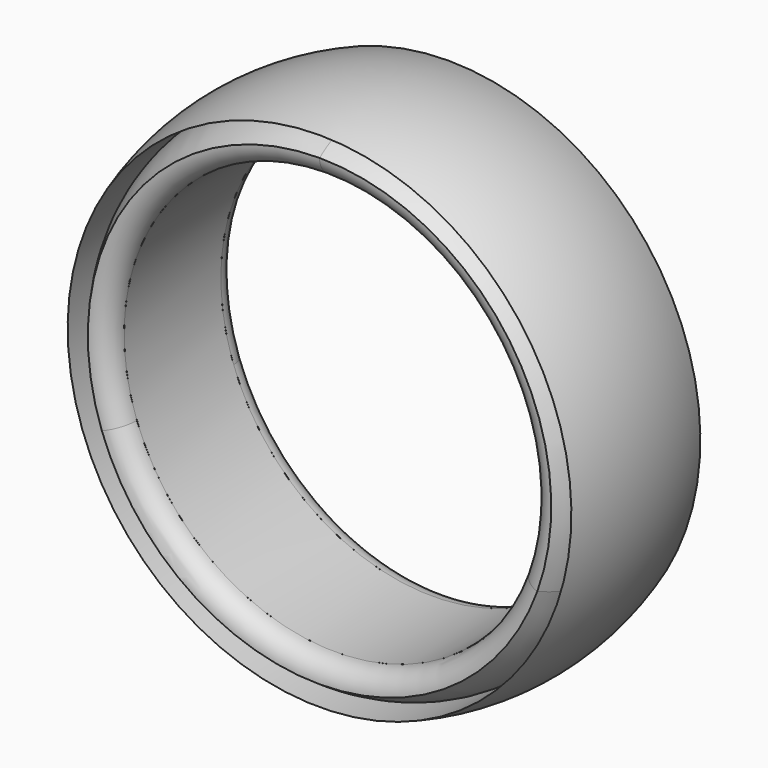
from build123d import *

# Parameters (mm, degrees)
F2_R           = 1
F3_ANGLE       = 110
F4_R           = 0.99999
F5_ANGLE_START = 110
F5_ANGLE       = 140
F6_R           = 0.99999
F7_ANGLE_START = 250
F7_ANGLE       = 110
F8_R           = 0.99999
F10_T2_ANGLE   = 208.8221013409
F10_T4_ANGLE   = 208.8221013409
F10_2_T2_ANGLE = 178.7965067315
F10_2_T4_ANGLE = 178.7965067315
F10_3_T2_ANGLE = 178.7965067315
F10_3_T4_ANGLE = 178.7965067315


# Not quite as in the source:
# - a fillet or chamfer that OpenCascade refuses, or shapes differently, is made with other operations: its cross-section is extruded or revolved along the edge and cut away or added
# - a fillet or chamfer is up to 0.001 mm smaller than in the source, because OpenCascade refuses the exact size


with BuildPart() as f1:
    # F0 (on Right) → F1 (revolve)
    with BuildSketch(Plane.YZ):
        Polygon((18.100000754, -6.0000002161), (18.100000754, -7.0000002161), (24.100000754, -7.0000002161), (24.100000754, -6.0000002161), (23.100000754, -6.0000002161), (22.7464473634, -5.6464468255), (19.4535541446, -5.6464468255), (19.100000754, -6.0000002161), align=None)
    revolve(axis=Axis((0, 30.3733862936, -17.5), (0, 1, 0)))

    # F2
    f2_edges = [f1.edges().sort_by_distance(p)[0] for p in [
        (0, 19.453554, -29.353553),
        (0, 22.746447, -29.353553),
    ]]
    fillet(f2_edges, radius=F2_R)


with BuildPart() as f3:
    # F0 (on Right) → F3 (revolve)
    with BuildSketch(Plane.YZ):
        Polygon((25.100000754, -5.0000002161), (17.100000754, -5.0000002161), (17.100000754, -7.0000002161), (18.100000754, -7.0000002161), (18.100000754, -6.0000002161), (19.100000754, -6.0000002161), (19.4535541446, -5.6464468255), (22.7464473634, -5.6464468255), (23.100000754, -6.0000002161), (24.100000754, -6.0000002161), (24.100000754, -7.0000002161), (25.100000754, -7.0000002161), (25.100000754, -6.0000002161), align=None)
    revolve(axis=Axis((0, 30.3733862936, -17.5), (0, 1, 0)), revolution_arc=F3_ANGLE)

    # F4 (radius 1 in the source; OpenCascade refuses exactly that, so slightly less here)
    f4_edges = [f3.edges().sort_by_distance(p)[0] for p in [
        (9.420248, 23.100001, -10.903871),
        (9.709862, 19.453554, -10.701081),
        (8.601096, 17.100001, -11.477448),
        (8.601096, 25.100001, -11.477448),
    ]]
    fillet(f4_edges, radius=F4_R)

    # F10#3: fillet of radius 5 on 2 edges, made by hand

    # F10_3_s1 → F10_3_t2 (revolve, cut)
    with BuildSketch(Plane(origin=(-8.1576403263, 0, -5.5852876424), x_dir=(0, 1, 0), z_dir=(-0.8251307206, 0, -0.56494185))):
        with BuildLine():
            ThreePointArc((22.0999874207, 1.9397878273), (23.6811341565, 2.1963739723), (25.100000754, 2.9397978273))
            Line((25.100000754, 2.9397978273), (25.1600010207, 2.8597980273))
            ThreePointArc((25.1600010207, 2.8597980273), (25.200000754, 2.4397928273), (25.200000754, 1.9397878273))
            Line((25.200000754, 1.9397878273), (25.100000754, 1.8397878273))
            Line((25.100000754, 1.8397878273), (22.0999874207, 1.8397878273))
            Line((22.0999874207, 1.8397878273), (22.0999874207, 1.9397878273))
        make_face()
    revolve(axis=Axis((0, 25.100000754, -17.5), (0, 1, 0)), revolution_arc=F10_3_T2_ANGLE, mode=Mode.SUBTRACT)

    # F10_3_s3 → F10_3_t4 (revolve, cut)
    with BuildSketch(Plane(origin=(-8.1576403263, 0, -5.5852876424), x_dir=(0, 1, 0), z_dir=(-0.8251307206, 0, -0.56494185))):
        with BuildLine():
            ThreePointArc((17.100000754, 2.9397978273), (18.5188673515, 2.1963739723), (20.1000140873, 1.9397878273))
            Line((20.1000140873, 1.9397878273), (20.1000140873, 1.8397878273))
            Line((20.1000140873, 1.8397878273), (17.100000754, 1.8397878273))
            Line((17.100000754, 1.8397878273), (17.000000754, 1.9397878273))
            ThreePointArc((17.000000754, 1.9397878273), (17.000000754, 2.4397928273), (17.0400004873, 2.8597980273))
            Line((17.0400004873, 2.8597980273), (17.100000754, 2.9397978273))
        make_face()
    revolve(axis=Axis((0, 17.100000754, -17.5), (0, 1, 0)), revolution_arc=F10_3_T4_ANGLE, mode=Mode.SUBTRACT)


with BuildPart() as f5:
    # F0 (on Right) → F5 (revolve)
    with BuildSketch(Plane.YZ, mode=Mode.PRIVATE) as f5_sk:
        Polygon((25.100000754, -5.0000002161), (17.100000754, -5.0000002161), (17.100000754, -7.0000002161), (18.100000754, -7.0000002161), (18.100000754, -6.0000002161), (19.100000754, -6.0000002161), (19.4535541446, -5.6464468255), (22.7464473634, -5.6464468255), (23.100000754, -6.0000002161), (24.100000754, -6.0000002161), (24.100000754, -7.0000002161), (25.100000754, -7.0000002161), (25.100000754, -6.0000002161), align=None)
    revolve(f5_sk.sketch.rotate(Axis((0, 30.3733862936, -17.5), (0, 1, 0)), F5_ANGLE_START), axis=Axis((0, 30.3733862936, -17.5), (0, 1, 0)), revolution_arc=F5_ANGLE)

    # F6 (radius 1 in the source; OpenCascade refuses exactly that, so slightly less here)
    f6_edges = [f5.edges().sort_by_distance(p)[0] for p in [
        (0, 23.100001, -29),
        (0, 25.100001, -28),
        (0, 17.100001, -28),
        (0, 19.453554, -29.353553),
    ]]
    fillet(f6_edges, radius=F6_R)

    # F10: fillet of radius 5 on 2 edges, made by hand

    # F10_s1 → F10_t2 (revolve, cut)
    with BuildSketch(Plane(origin=(4.2183020759, 0, -16.416056848), x_dir=(0, 1, 0), z_dir=(-0.2488766937, 0, 0.9685351781))):
        with BuildLine():
            ThreePointArc((22.0999874207, -8.1446576435), (23.6811341565, -7.8880714985), (25.100000754, -7.1446476435))
            Line((25.100000754, -7.1446476435), (25.1600010207, -7.2246474435))
            ThreePointArc((25.1600010207, -7.2246474435), (25.200000754, -7.6446526435), (25.200000754, -8.1446576435))
            Line((25.200000754, -8.1446576435), (25.100000754, -8.2446576435))
            Line((25.100000754, -8.2446576435), (22.0999874207, -8.2446576435))
            Line((22.0999874207, -8.2446576435), (22.0999874207, -8.1446576435))
        make_face()
    revolve(axis=Axis((0, 25.100000754, -17.5), (0, 1, 0)), revolution_arc=F10_T2_ANGLE, mode=Mode.SUBTRACT)

    # F10_s3 → F10_t4 (revolve, cut)
    with BuildSketch(Plane(origin=(4.2183020759, 0, -16.416056848), x_dir=(0, 1, 0), z_dir=(-0.2488766937, 0, 0.9685351781))):
        with BuildLine():
            ThreePointArc((17.100000754, -7.1446476435), (18.5188673515, -7.8880714985), (20.1000140873, -8.1446576435))
            Line((20.1000140873, -8.1446576435), (20.1000140873, -8.2446576435))
            Line((20.1000140873, -8.2446576435), (17.100000754, -8.2446576435))
            Line((17.100000754, -8.2446576435), (17.000000754, -8.1446576435))
            ThreePointArc((17.000000754, -8.1446576435), (17.000000754, -7.6446526435), (17.0400004873, -7.2246474435))
            Line((17.0400004873, -7.2246474435), (17.100000754, -7.1446476435))
        make_face()
    revolve(axis=Axis((0, 17.100000754, -17.5), (0, 1, 0)), revolution_arc=F10_T4_ANGLE, mode=Mode.SUBTRACT)


with BuildPart() as f7:
    # F0 (on Right) → F7 (revolve)
    with BuildSketch(Plane.YZ, mode=Mode.PRIVATE) as f7_sk:
        Polygon((25.100000754, -5.0000002161), (17.100000754, -5.0000002161), (17.100000754, -7.0000002161), (18.100000754, -7.0000002161), (18.100000754, -6.0000002161), (19.100000754, -6.0000002161), (19.4535541446, -5.6464468255), (22.7464473634, -5.6464468255), (23.100000754, -6.0000002161), (24.100000754, -6.0000002161), (24.100000754, -7.0000002161), (25.100000754, -7.0000002161), (25.100000754, -6.0000002161), align=None)
    revolve(f7_sk.sketch.rotate(Axis((0, 30.3733862936, -17.5), (0, 1, 0)), F7_ANGLE_START), axis=Axis((0, 30.3733862936, -17.5), (0, 1, 0)), revolution_arc=F7_ANGLE)

    # F8 (radius 1 in the source; OpenCascade refuses exactly that, so slightly less here)
    f8_edges = [f7.edges().sort_by_distance(p)[0] for p in [
        (-9.709862, 19.453554, -10.701081),
        (-8.601096, 17.100001, -11.477448),
        (-8.601096, 25.100001, -11.477448),
        (-9.420248, 23.100001, -10.903871),
    ]]
    fillet(f8_edges, radius=F8_R)

    # F10#2: fillet of radius 5 on 2 edges, made by hand

    # F10_2_s1 → F10_2_t2 (revolve, cut)
    with BuildSketch(Plane(origin=(8.2833529326, 0, -5.9306801895), x_dir=(0, 1, 0), z_dir=(0.8130830149, 0, -0.5821477569))):
        with BuildLine():
            ThreePointArc((17.100000754, -25.7289425452), (18.5188673515, -26.4723664002), (20.1000140873, -26.7289525452))
            Line((20.1000140873, -26.7289525452), (20.1000140873, -26.8289525452))
            Line((20.1000140873, -26.8289525452), (17.100000754, -26.8289525452))
            Line((17.100000754, -26.8289525452), (17.000000754, -26.7289525452))
            ThreePointArc((17.000000754, -26.7289525452), (17.000000754, -26.2289475452), (17.0400004873, -25.8089423452))
            Line((17.0400004873, -25.8089423452), (17.100000754, -25.7289425452))
        make_face()
    revolve(axis=Axis((0, 17.100000754, -17.5), (0, 1, 0)), revolution_arc=F10_2_T2_ANGLE, mode=Mode.SUBTRACT)

    # F10_2_s3 → F10_2_t4 (revolve, cut)
    with BuildSketch(Plane(origin=(8.2833529326, 0, -5.9306801895), x_dir=(0, 1, 0), z_dir=(0.8130830149, 0, -0.5821477569))):
        with BuildLine():
            ThreePointArc((22.0999874207, -26.7289525452), (23.6811341565, -26.4723664002), (25.100000754, -25.7289425452))
            Line((25.100000754, -25.7289425452), (25.1600010207, -25.8089423452))
            ThreePointArc((25.1600010207, -25.8089423452), (25.200000754, -26.2289475452), (25.200000754, -26.7289525452))
            Line((25.200000754, -26.7289525452), (25.100000754, -26.8289525452))
            Line((25.100000754, -26.8289525452), (22.0999874207, -26.8289525452))
            Line((22.0999874207, -26.8289525452), (22.0999874207, -26.7289525452))
        make_face()
    revolve(axis=Axis((0, 25.100000754, -17.5), (0, 1, 0)), revolution_arc=F10_2_T4_ANGLE, mode=Mode.SUBTRACT)


with BuildPart() as f9:
    # F0 (on Right) → F9 (revolve)
    with BuildSketch(Plane.YZ):
        with BuildLine():
            ThreePointArc((25.100000754, -5.0000002161), (21.100000754, -4.3563002289), (17.100000754, -5.0000002161))
            Line((17.100000754, -5.0000002161), (25.100000754, -5.0000002161))
        make_face()
    revolve(axis=Axis((0, 6.3473723829, -17.5), (0, 1, 0)))


solid = Compound([f1.part, f3.part, f5.part, f7.part, f9.part])
